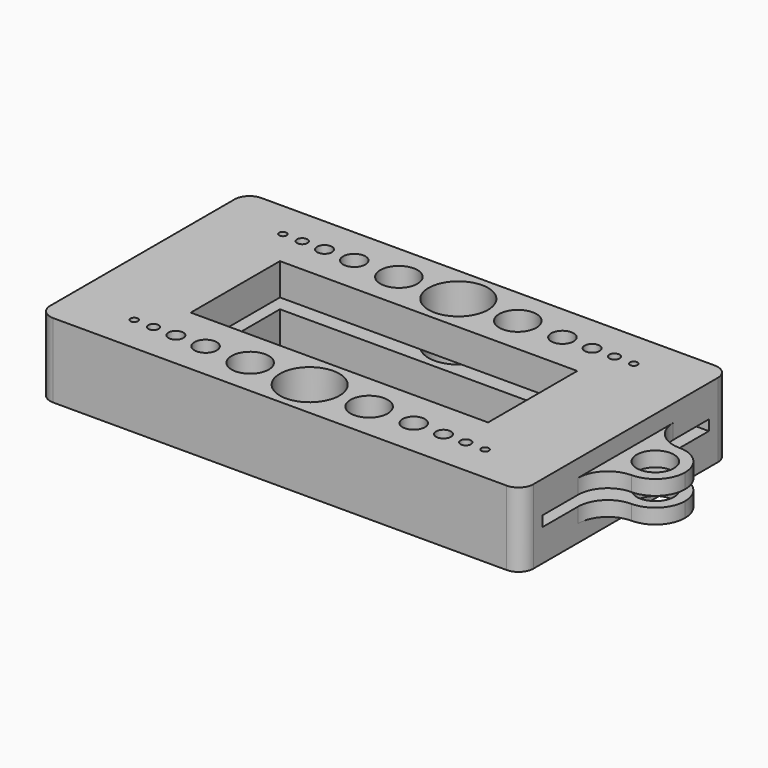
from build123d import *

# Parameters (mm, degrees)
F1_DEPTH  = 6.35
F2_W      = 50.8
F2_H      = 19.05
F2_R      = 5.08
F2_R_2    = 3.175
F2_R_3    = 0.635
F2_R_4    = 1.905
F2_R_5    = 1.27
F2_R_6    = 0.889
F3_DEPTH  = 12.7
F4_W      = 35.56
F4_H      = 1.778
F5_DEPTH  = 76.2
F6_W      = 10.16
F6_H      = 2.54
F7_DEPTH  = 10.16
F8_R      = 5.07999
F9_R      = 3.175
F10_DEPTH = 25.4


# Not quite as in the source:
# - a fillet or chamfer is up to 0.001 mm smaller than in the source, because OpenCascade refuses the exact size


with BuildPart() as f1:
    # F0 (on Top) → F1 (new body, symmetric)
    with BuildSketch(Plane.XY):
        with BuildLine():
            Line((38.735, 22.225), (-38.735, 22.225))
            ThreePointArc((-38.735, 22.225), (-40.5310512242, 21.4810512242), (-41.275, 19.685))
            Line((-41.275, 19.685), (-41.275, -19.685))
            ThreePointArc((-41.275, -19.685), (-40.5310512242, -21.4810512242), (-38.735, -22.225))
            Line((-38.735, -22.225), (38.735, -22.225))
            ThreePointArc((38.735, -22.225), (40.5310512242, -21.4810512242), (41.275, -19.685))
            Line((41.275, -19.685), (41.275, 19.685))
            ThreePointArc((41.275, 19.685), (40.5310512242, 21.4810512242), (38.735, 22.225))
        make_face()
    extrude(amount=F1_DEPTH, both=True)

    # F2 (on face) → F3 (cut, through all)
    with BuildSketch(Plane.XY.offset(6.35)):
        Rectangle(F2_W, F2_H)
        with Locations((0, 15.875)):
            Circle(F2_R)
        with Locations((-10.16, 15.875)):
            Circle(F2_R_2)
        with Locations((-29.972, 15.875)):
            Circle(F2_R_3)
        with Locations((-17.78, 15.875)):
            Circle(F2_R_4)
        with Locations((-22.86, 15.875)):
            Circle(F2_R_5)
        with Locations((-26.67, 15.875)):
            Circle(F2_R_6)
        with Locations((29.972, 15.875)):
            Circle(F2_R_3)
        with Locations((22.86, 15.875)):
            Circle(F2_R_5)
        with Locations((26.67, 15.875)):
            Circle(F2_R_6)
        with Locations((17.78, 15.875)):
            Circle(F2_R_4)
        with Locations((10.16, 15.875)):
            Circle(F2_R_2)
        with Locations((29.972, -15.875)):
            Circle(F2_R_3)
        with Locations((0, -15.875)):
            Circle(F2_R)
        with Locations((26.67, -15.875)):
            Circle(F2_R_6)
        with Locations((-22.86, -15.875)):
            Circle(F2_R_5)
        with Locations((-29.972, -15.875)):
            Circle(F2_R_3)
        with Locations((22.86, -15.875)):
            Circle(F2_R_5)
        with Locations((17.78, -15.875)):
            Circle(F2_R_4)
        with Locations((-26.67, -15.875)):
            Circle(F2_R_6)
        with Locations((-10.16, -15.875)):
            Circle(F2_R_2)
        with Locations((10.16, -15.875)):
            Circle(F2_R_2)
        with Locations((-17.78, -15.875)):
            Circle(F2_R_4)
    extrude(amount=-F3_DEPTH, mode=Mode.SUBTRACT)

    # F4 (on face) → F5 (cut)
    with BuildSketch(Plane.YZ.offset(41.275)):
        Rectangle(F4_W, F4_H)
    extrude(amount=-F5_DEPTH, mode=Mode.SUBTRACT)

    # F6 (on face) → F7 (join)
    with BuildSketch(Plane.YZ.offset(41.275)):
        with Locations((0, 2.159)):
            Rectangle(F6_W, F6_H)
        with Locations((0, -2.159)):
            Rectangle(F6_W, F6_H)
    extrude(amount=F7_DEPTH)

    # F8 (radius 5.08 in the source; OpenCascade refuses exactly that, so slightly less here)
    f8_edges = [f1.edges().sort_by_distance(p)[0] for p in [
        (51.435, -5.08, 2.159),
        (51.435, 5.08, 2.159),
        (51.435, 5.08, -2.159),
        (51.435, -5.08, -2.159),
        (41.275, -5.08, 2.159),
        (41.275, -5.08, -2.159),
        (41.275, 5.08, 2.159),
        (41.275, 5.08, -2.159),
    ]]
    fillet(f8_edges, radius=F8_R)

    # F9 (on face) → F10 (cut)
    with BuildSketch(Plane.XY.offset(3.429)):
        with Locations((46.355, 0)):
            Circle(F9_R)
    extrude(amount=-F10_DEPTH, mode=Mode.SUBTRACT)


solid = f1.part
